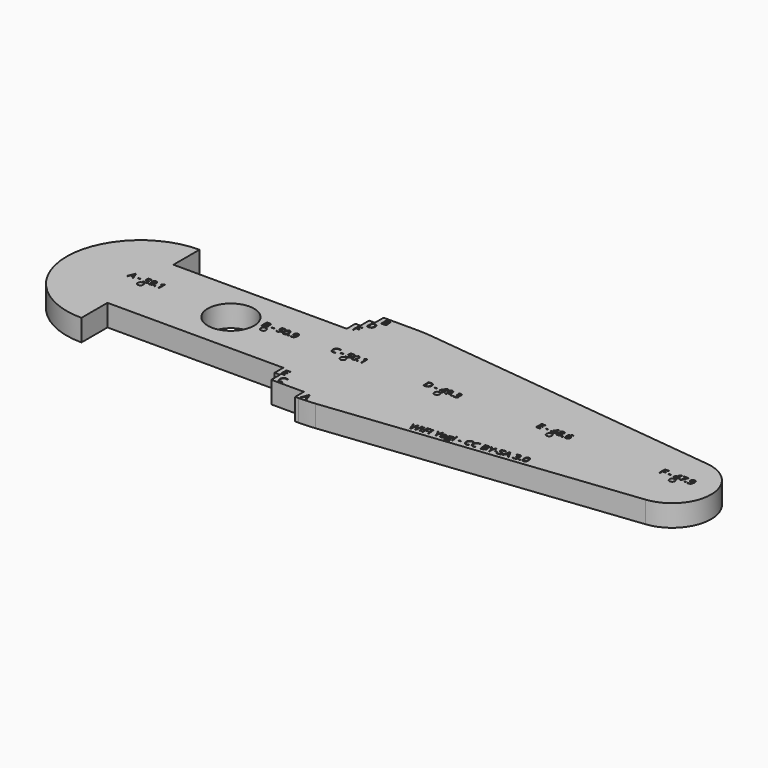
from build123d import *

# Parameters (mm, degrees)
F0_R         = 0.75
F0_R_2       = 6.4
F1_DEPTH     = 6
F2_TEXT_SIZE = 2.7777777778
F3_DEPTH     = 1
F4_TEXT_SIZE = 2.7777777778
F5_DEPTH     = 1
F6_DEPTH     = 5.001


# Not quite as in the source:
# - Text() gives the source's letters only with a copy of the font that has no kerning and outlines rounded to 1/6400 em; it was checked with that copy


with BuildPart() as f1:
    # F0 (on Top) → F1 (new body)
    with BuildSketch(Plane.XY):
        with BuildLine():
            Line((35, 20.4), (-25, 20.4))
            ThreePointArc((-25, 20.4), (-45.4, 0), (-25, -20.4))
            Line((-25, -20.4), (35, -20.4))
            ThreePointArc((35, -20.4), (37.2504805924, -20.3366415351), (39.4938318349, -20.1467668552))
            Line((39.4938318349, -20.1467668552), (123.2077173056, -10.6819435923))
            ThreePointArc((123.2077173056, -10.6819435923), (132.75, 0), (123.2077173056, 10.6819435923))
            Line((123.2077173056, 10.6819435923), (39.4938318349, 20.1467668552))
            ThreePointArc((39.4938318349, 20.1467668552), (37.2504805924, 20.3366415351), (35, 20.4))
        make_face()
        with Locations((-25, 0)):
            Circle(F0_R, mode=Mode.SUBTRACT)
        Circle(F0_R_2, mode=Mode.SUBTRACT)
        with Locations((9, 0)):
            Circle(F0_R, mode=Mode.SUBTRACT)
        with Locations((31, 0)):
            Circle(F0_R, mode=Mode.SUBTRACT)
        with Locations((57, 0)):
            Circle(F0_R, mode=Mode.SUBTRACT)
        with Locations((88, 0)):
            Circle(F0_R, mode=Mode.SUBTRACT)
        with Locations((122, 0)):
            Circle(F0_R, mode=Mode.SUBTRACT)
    extrude(amount=F1_DEPTH)

    # F2 (on face) → F3 (cut)
    with BuildSketch(Plane.XY.offset(6)):
        Polygon((25.9, 17.4), (25.9, 20.4), (-25, 20.4), (-25, 11.4), (22.9, 11.4), (22.9, 14.4), (24.3, 14.4), (24.3, 17.4), align=None)
        Polygon((-25, -11.4), (-25, -20.4), (34.1, -20.4), (34.1, -17.4), (25.1, -17.4), (25.1, -14.4), (23.6, -14.4), (23.6, -11.4), align=None)
        with Locations((-29.580078125, 1)):
            Text('A - 59.1', F2_TEXT_SIZE, font='Open Sans', text_align=(TextAlign.LEFT, TextAlign.BOTTOM))
        with Locations((7.3321211119, 1)):
            Text('B - 50.9', F2_TEXT_SIZE, font='Open Sans', text_align=(TextAlign.LEFT, TextAlign.BOTTOM))
        with Locations((26.4225260417, 1)):
            Text('C - 50.1', F2_TEXT_SIZE, font='Open Sans', text_align=(TextAlign.LEFT, TextAlign.BOTTOM))
        with Locations((52.0583767361, 1)):
            Text('D - 49.3', F2_TEXT_SIZE, font='Open Sans', text_align=(TextAlign.LEFT, TextAlign.BOTTOM))
        with Locations((83.2849392361, 1)):
            Text('E - 48.6', F2_TEXT_SIZE, font='Open Sans', text_align=(TextAlign.LEFT, TextAlign.BOTTOM))
        with Locations((117.3472222222, 1)):
            Text('F - 47.9', F2_TEXT_SIZE, font='Open Sans', text_align=(TextAlign.LEFT, TextAlign.BOTTOM))
        with Locations((23.9, 11.9)):
            Text('F', F2_TEXT_SIZE, font='Open Sans', text_align=(TextAlign.LEFT, TextAlign.BOTTOM))
        with Locations((26.9, 17.9)):
            Text('B', F2_TEXT_SIZE, font='Open Sans', text_align=(TextAlign.LEFT, TextAlign.BOTTOM))
        with Locations((25.3, 14.9)):
            Text('D', F2_TEXT_SIZE, font='Open Sans', text_align=(TextAlign.LEFT, TextAlign.BOTTOM))
        with Locations((24.6, -13.9)):
            Text('E', F2_TEXT_SIZE, font='Open Sans', text_align=(TextAlign.LEFT, TextAlign.BOTTOM))
        with Locations((26.1, -16.9)):
            Text('C', F2_TEXT_SIZE, font='Open Sans', text_align=(TextAlign.LEFT, TextAlign.BOTTOM))
        with Locations((35.1, -19.9)):
            Text('A', F2_TEXT_SIZE, font='Open Sans', text_align=(TextAlign.LEFT, TextAlign.BOTTOM))
    extrude(amount=-F3_DEPTH, mode=Mode.SUBTRACT)

    # F4 (on face) → F5 (cut)
    with BuildSketch(Plane.XY.offset(6)):
        with Locations(Location((62.1143071575, -16.4346292215), (0, 0, 6.4505581629))):
            Text('WIFI Yagi - CC BY-SA 3.0', F4_TEXT_SIZE, font='Open Sans', text_align=(TextAlign.LEFT, TextAlign.BOTTOM))
    extrude(amount=-F5_DEPTH, mode=Mode.SUBTRACT)

    # F6 (cut, through all): faces of the model
    f6_faces = [f1.faces().sort_by_distance(p)[0] for p in [
        (-0.3014517218, 15.9607697502, 5),
        (1.5043726236, -16.0996197719, 5),
    ]]
    extrude(f6_faces, amount=-F6_DEPTH, mode=Mode.SUBTRACT)


solid = f1.part
